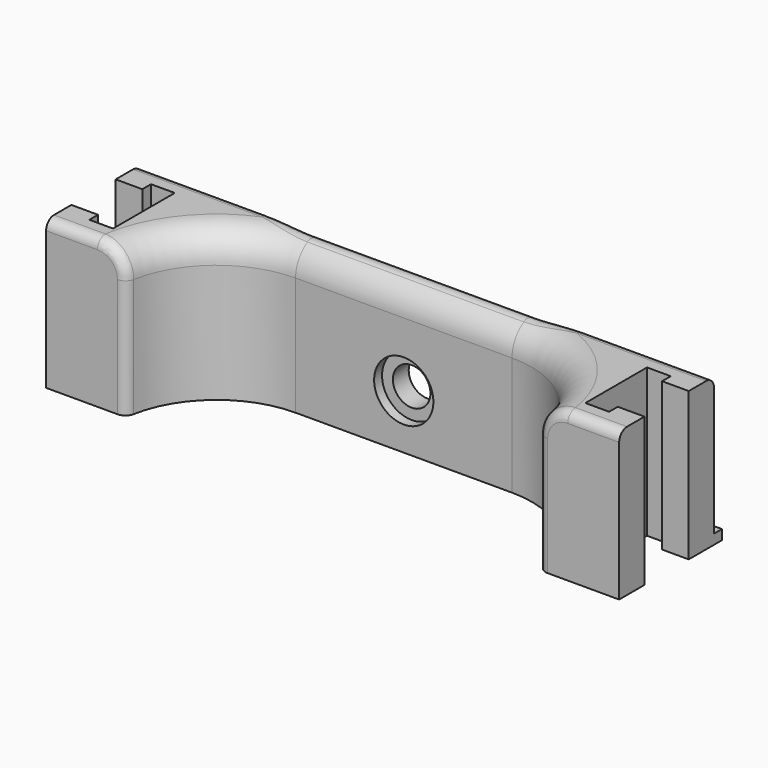
from build123d import *

# Parameters (mm, degrees)
F0_W           = 58
F0_H           = 15
F2_DEPTH       = 12
F4_DEPTH       = 25
F5_W           = 41.8
F5_H           = 9
F6_DEPTH       = 25
F1_W           = 58
F1_H           = 1
F8_DEPTH       = 1
F9_D           = 3.8
F9_CBORE_D     = 6
F9_CBORE_DEPTH = 1
F10_T1_DEPTH   = 15
F11_R          = 2.99999
F12_R          = 1
F13_R          = 1


# Not quite as in the source:
# - a fillet or chamfer that OpenCascade refuses, or shapes differently, is made with other operations: its cross-section is extruded or revolved along the edge and cut away or added
# - a fillet or chamfer is up to 0.001 mm smaller than in the source, because OpenCascade refuses the exact size


with BuildPart() as f2:
    # F0 (on Front) → F2 (new body)
    with BuildSketch(Plane.XZ):
        with Locations((0, 7.5)):
            Rectangle(F0_W, F0_H)
    extrude(amount=F2_DEPTH)

    # F3 (on Top) → F4 (cut)
    with BuildSketch(Plane.XY):
        Polygon((-26.3, -3.2), (-29, -3.2), (-29, -8.8), (-26.3, -8.8), (-26.3, -9.9), (-23.9, -9.9), (-23.9, -2.1), (-26.3, -2.1), align=None)
        Polygon((29, -8.8), (29, -3.2), (26.3, -3.2), (26.3, -2.1), (23.9, -2.1), (23.9, -9.9), (26.3, -9.9), (26.3, -8.8), align=None)
    extrude(amount=F4_DEPTH, mode=Mode.SUBTRACT)

    # F5 (on Top) → F6 (cut)
    with BuildSketch(Plane.XY):
        with Locations((0, -7.5)):
            Rectangle(F5_W, F5_H)
    extrude(amount=F6_DEPTH, mode=Mode.SUBTRACT)

    # F1 (on Front) → F8 (join)
    with BuildSketch(Plane.XZ):
        with Locations((0, 0.5)):
            Rectangle(F1_W, F1_H)
    extrude(amount=-F8_DEPTH)

    # F9 (through all)
    with Locations(Plane.XZ.offset(3)):
        with Locations((0, 5.5)):
            CounterBoreHole(F9_D / 2, F9_CBORE_D / 2, F9_CBORE_DEPTH)

    # F10: fillet of radius 10 on 2 edges, made by hand

    # F10_s2 → F10_t1 (join)
    with BuildSketch(Plane.XY):
        with BuildLine():
            ThreePointArc((-20.9, -12), (-17.6583295614, -5.5838015129), (-10.9501256289, -3))
            Line((-10.9501256289, -3), (-20.9, -3))
            Line((-20.9, -3), (-20.9, -12))
        make_face()
        with BuildLine():
            ThreePointArc((10.9501256289, -3), (17.6583295614, -5.5838015129), (20.9, -12))
            Line((20.9, -12), (20.9, -3))
            Line((20.9, -3), (10.9501256289, -3))
        make_face()
    extrude(amount=F10_T1_DEPTH)

    # F11 (radius 3 in the source; OpenCascade refuses exactly that, so slightly less here)
    f11_edges = [f2.edges().sort_by_distance(p)[0] for p in [
        (0, -3, 15),
        (17.65833, -5.583802, 15),
        (-17.65833, -5.583802, 15),
    ]]
    fillet(f11_edges, radius=F11_R)

    # F12
    f12_edges = [f2.edges().sort_by_distance(p)[0] for p in [
        (-26.455798, -12, 15),
        (26.455798, -12, 15),
    ]]
    fillet(f12_edges, radius=F12_R)

    # F13
    f13_edges = [f2.edges().sort_by_distance(p)[0] for p in [
        (0, 0, 15),
    ]]
    fillet(f13_edges, radius=F13_R)


solid = f2.part
